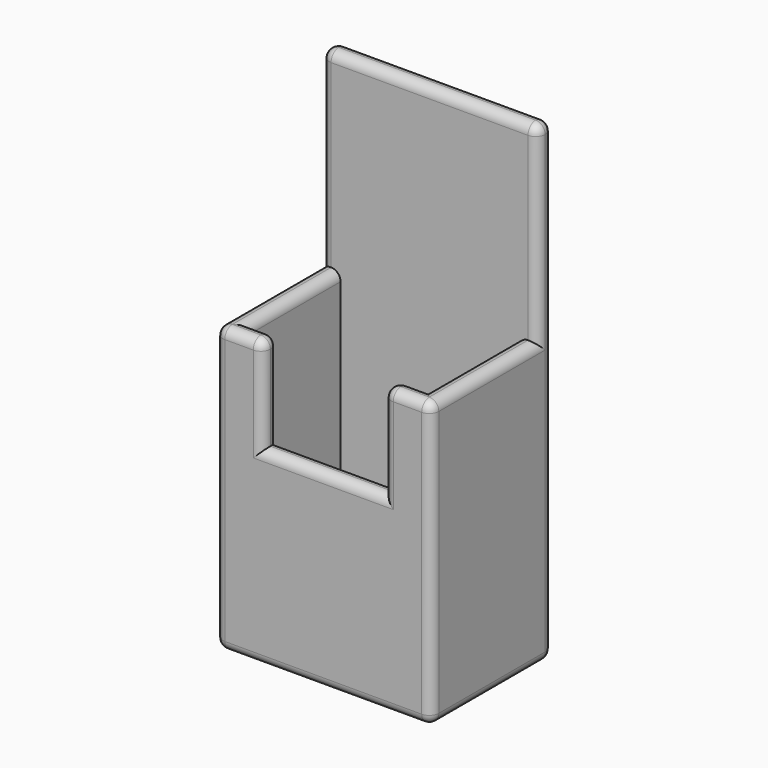
from build123d import *

# Parameters (mm, degrees)
F1_DEPTH = 5.08
F0_W     = 32.385
F0_H     = 5.08
F2_DEPTH = 50.8
F3_DEPTH = 76.2
F4_DEPTH = 127
F5_R     = 2.53999


# Not quite as in the source:
# - a fillet or chamfer is up to 0.001 mm smaller than in the source, because OpenCascade refuses the exact size


with BuildPart() as f1:
    # F0 (on Top) → F1 (new body)
    with BuildSketch(Plane.XY):
        Polygon((23.8125, 15.24), (-23.8125, 15.24), (-23.8125, -15.24), (-16.1925, -15.24), (16.1925, -15.24), (23.8125, -15.24), align=None)
    extrude(amount=F1_DEPTH)

    # F0 (on Top) → F2 (join)
    with BuildSketch(Plane.XY):
        with Locations((0, -17.78)):
            Rectangle(F0_W, F0_H)
    extrude(amount=F2_DEPTH)

    # F0 (on Top) → F3 (join)
    with BuildSketch(Plane.XY):
        Polygon((-23.8125, 15.24), (-28.8925, 15.24), (-28.8925, -20.32), (-16.1925, -20.32), (-16.1925, -15.24), (-23.8125, -15.24), align=None)
        Polygon((28.8925, -20.32), (28.8925, 15.24), (23.8125, 15.24), (23.8125, -15.24), (16.1925, -15.24), (16.1925, -20.32), align=None)
    extrude(amount=F3_DEPTH)

    # F0 (on Top) → F4 (join)
    with BuildSketch(Plane.XY):
        Polygon((28.8925, 20.32), (-28.8925, 20.32), (-28.8925, 15.24), (-23.8125, 15.24), (23.8125, 15.24), (28.8925, 15.24), align=None)
    extrude(amount=F4_DEPTH)

    # F5 (radius 2.54 in the source; OpenCascade refuses exactly that, so slightly less here)
    f5_edges = [f1.edges().sort_by_distance(p)[0] for p in [
        (28.8925, -20.32, 38.1),
        (22.5425, -20.32, 76.2),
        (16.1925, -20.32, 63.5),
        (0, -20.32, 50.8),
        (-16.1925, -20.32, 63.5),
        (-22.5425, -20.32, 76.2),
        (-28.8925, -20.32, 38.1),
        (0, -20.32, 0),
        (-16.1925, -15.24, 63.5),
        (0, -15.24, 50.8),
        (-20.0025, -15.24, 76.2),
        (20.0025, -15.24, 76.2),
        (16.1925, -15.24, 63.5),
        (16.1925, -17.78, 76.2),
        (-16.1925, -17.78, 76.2),
        (23.8125, 0, 76.2),
        (-23.8125, 0, 76.2),
        (28.8925, -2.54, 76.2),
        (28.8925, 15.24, 101.6),
        (28.8925, 17.78, 127),
        (28.8925, 20.32, 63.5),
        (28.8925, 0, 0),
        (0, 15.24, 127),
        (-28.8925, 15.24, 101.6),
        (0, 20.32, 127),
        (-28.8925, 20.32, 63.5),
        (-28.8925, -2.54, 76.2),
        (-28.8925, 0, 0),
        (0, 20.32, 0),
        (-28.8925, 17.78, 127),
    ]]
    fillet(f5_edges, radius=F5_R)


solid = f1.part
